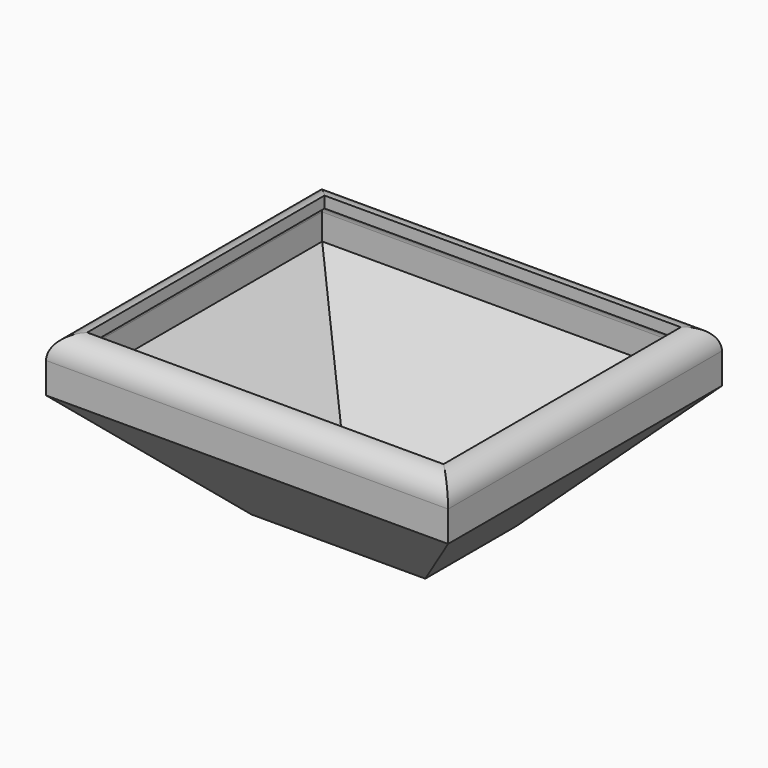
from build123d import *

# Parameters (mm, degrees)
F0_W     = 89.4973501563
F0_H     = 37.3169183731
F1_DEPTH = 76.2
F2_R     = 5.08
F3_SIZE  = 25.4
F4_T     = -2.54
F6_D     = 6.35


# Not quite as in the source:
# - a shell that OpenCascade refuses in one call is made with other operations: the cavity is built on its own and cut out


with BuildPart() as f1:
    # F0 (on Front) → F1 (new body)
    with BuildSketch(Plane.XZ):
        with Locations((0.0334233046, 18.6584591866)):
            Rectangle(F0_W, F0_H)
    extrude(amount=F1_DEPTH)

    # F2
    f2_edges = [f1.edges().sort_by_distance(p)[0] for p in [
        (44.782098, -38.1, 37.316918),
        (0.033423, -76.2, 37.316918),
        (-44.715252, -38.1, 37.316918),
        (0.033423, 0, 37.316918),
    ]]
    fillet(f2_edges, radius=F2_R)

    # F3
    f3_edges = [f1.edges().sort_by_distance(p)[0] for p in [
        (-44.715252, -38.1, 0),
        (0.033423, 0, 0),
        (44.782098, -38.1, 0),
        (0.033423, -76.2, 0),
    ]]
    chamfer(f3_edges, length=F3_SIZE)

    # F4: a shell. OpenCascade refuses it in one call, so the cavity is built on its own and cut out:
    # the body offset inwards by the wall thickness, plus a prism from it out through each open face.
    f4_core = offset(f1.part, amount=F4_T, mode=Mode.PRIVATE)
    f4_exits = [f4_core.faces().sort_by_distance(p)[0] for p in [
        (0.033423, -38.1, 34.776918),
    ]]
    add(f4_core, mode=Mode.SUBTRACT)
    extrude(f4_exits, amount=-F4_T, mode=Mode.SUBTRACT)

    # F6 (through all)
    with Locations(Plane.XY.offset(2.54)):
        with Locations((0.0334233046, -40.5182316899)):
            Hole(F6_D / 2)


solid = f1.part
